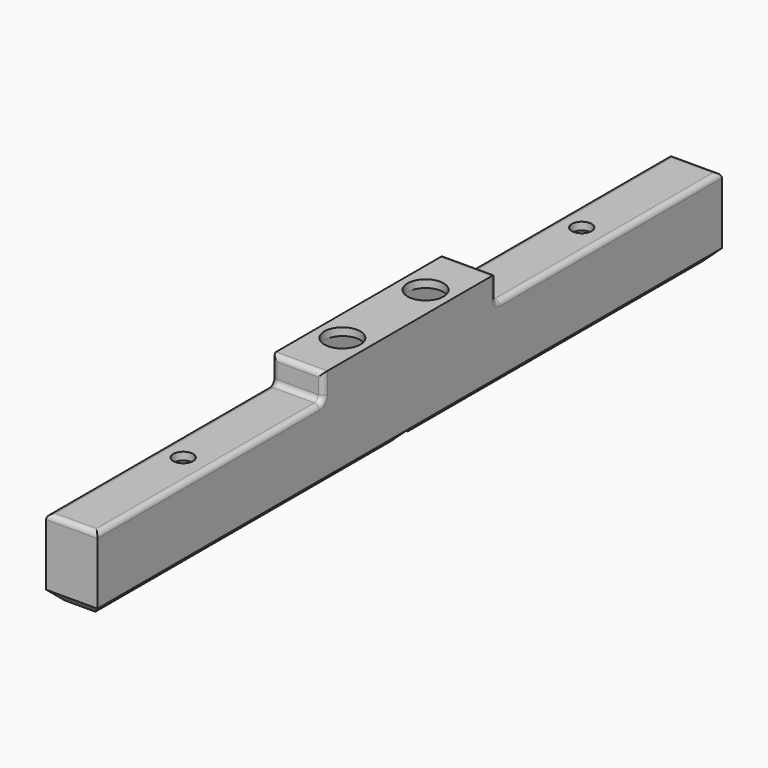
from build123d import *

# Parameters (mm, degrees)
F1_DEPTH       = 25.4
F2_F1_R        = 2.54
F2_F2_R        = 2.54
F3_SIZE        = 5.08
F4_T           = -3.81
F5_R           = 8.89
F6_DEPTH       = 3.81
F7_D           = 5.5
F7_DEPTH       = 12.7
F7_START       = 12.7
F7_CBORE_D     = 9.75
F7_CBORE_DEPTH = 5
F7_TIP         = 1.6523667023


with BuildPart() as f1:
    # F0 (on Right) → F1 (new body)
    with BuildSketch(Plane.YZ):
        Polygon((-190.5, 60.4147898585), (-243.84, 60.4147898585), (-243.84, 9.6147898585), (-50.8, 9.6147898585), (-50.8, 47.7147898585), (-190.5, 47.7147898585), align=None)
    extrude(amount=F1_DEPTH)

    # F2: fillet of radius 2.54 on 5 edges, made by hand

    # F2_f1
    f2_f1_edges = [f1.edges().sort_by_distance(p)[0] for p in [
        (12.7, -190.5, 47.7147898585),
    ]]
    fillet(f2_f1_edges, radius=F2_F1_R)

    # F2_f2
    f2_f2_edges = [f1.edges().sort_by_distance(p)[0] for p in [
        (25.4, -119.38, 47.7147898585),
        (0, -119.38, 47.7147898585),
        (12.7, -50.8, 47.7147898585),
        (12.7, -190.5, 60.4147898585),
        (0, -189.7560512242, 48.4587386342),
        (25.4, -189.7560512242, 48.4587386342),
    ]]
    fillet(f2_f2_edges, radius=F2_F2_R)

    # F3
    f3_edges = [f1.edges().sort_by_distance(p)[0] for p in [
        (25.4, -147.32, 9.61479),
        (12.7, -243.84, 9.61479),
        (12.7, -50.8, 9.61479),
        (0, -147.32, 9.61479),
    ]]
    chamfer(f3_edges, length=F3_SIZE)

    # F4
    f4_openings = [f1.faces().sort_by_distance(p)[0] for p in [
        (12.7, -243.84, 37.55479),
    ]]
    offset(amount=F4_T, openings=f4_openings)

    # F5 (on face) → F6 (cut, through all)
    with BuildSketch(Plane.XY.offset(60.4147898585)):
        with Locations((12.7, -218.1196852207)):
            Circle(F5_R)
    extrude(amount=-F6_DEPTH, mode=Mode.SUBTRACT)

    # F7
    # its depths count from where the whole tool has entered the part; down to there all is cleared
    with Locations(Plane.XY.offset(60.4147898585).offset(-F7_START)):
        with Locations((11.946093291, -120.65)):
            CounterBoreHole(F7_D / 2, F7_CBORE_D / 2, F7_CBORE_DEPTH, depth=F7_DEPTH)
            with Locations((0, 0, -(F7_DEPTH + F7_TIP / 2))):  # 118° drill point
                Cone(0, F7_D / 2, F7_TIP, mode=Mode.SUBTRACT)

    # F8: F1 across face


with BuildPart() as f1_1:
    add(f1.part)
    add(f1.part.mirror(Plane(origin=(12.7, -243.84, 36.5538832465), x_dir=(1, 0, 0), z_dir=(0, -1, 0))))


solid = f1_1.part
